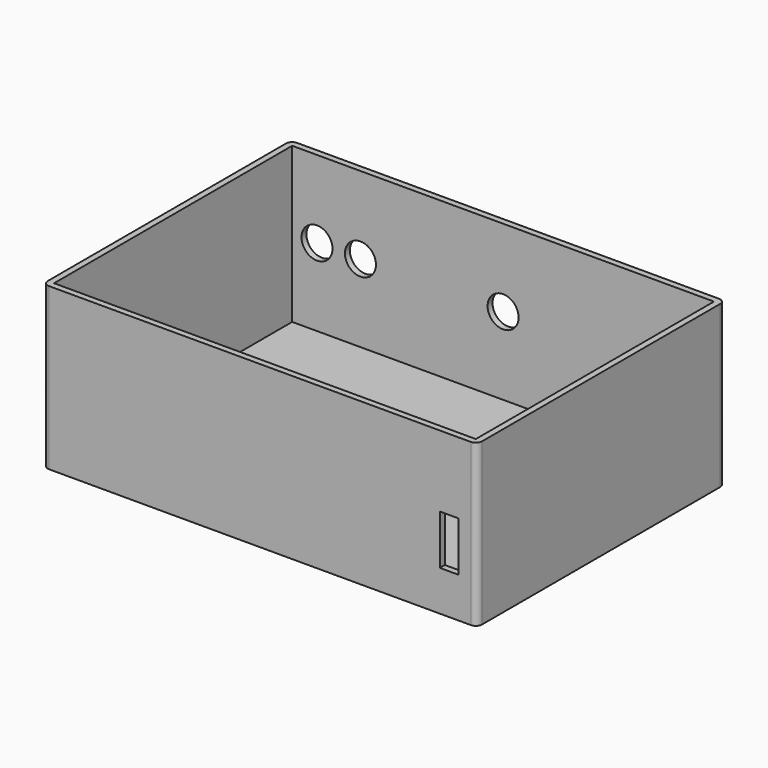
from build123d import *

# Parameters (mm, degrees)
F0_W          = 70
F0_H          = 50
F1_DEPTH      = 1
F2_W          = 70
F2_H          = 50
F2_W_2        = 68
F2_H_2        = 48
F3_DEPTH      = 25
F4_R          = 1
F5_W          = 3
F5_H          = 8
F6_DEPTH      = 25
F7_W          = 5
F7_H          = 10
F8_DEPTH      = 25
F9_R          = 2.5
F10_DEPTH     = 25
F11_R         = 2.5
F12_DEPTH     = 25
F13_R         = 2.5
F14_DEPTH     = 25
F15_TEXT_SIZE = 6.9444444444
F16_DEPTH     = 0.5


# Not quite as in the source:
# - Text() gives the source's letters only with a copy of the font that has no kerning and outlines rounded to 1/6400 em; it was checked with that copy


with BuildPart() as f1:
    # F0 (on Top) → F1 (new body)
    with BuildSketch(Plane.XY):
        with Locations((0, -0.7945728756)):
            Rectangle(F0_W, F0_H)
    extrude(amount=F1_DEPTH)

    # F2 (on face) → F3 (join)
    with BuildSketch(Plane.XY.offset(1)):
        with Locations((0, -0.7945728756)):
            Rectangle(F2_W, F2_H)
        with Locations((0, -0.7945728756)):
            Rectangle(F2_W_2, F2_H_2, mode=Mode.SUBTRACT)
    extrude(amount=F3_DEPTH)

    # F4
    f4_edges = [f1.edges().sort_by_distance(p)[0] for p in [
        (-35, 24.205427, 13),
        (-35, -25.794573, 13),
        (35, 24.205427, 13),
        (35, -25.794573, 13),
    ]]
    fillet(f4_edges, radius=F4_R)

    # F5 (on face) → F6 (cut)
    with BuildSketch(Plane(origin=(0, -24.7945728756, 0), x_dir=(-1, 0, 0), z_dir=(0, 1, 0))):
        with Locations((-30.5, 10.5)):
            Rectangle(F5_W, F5_H)
    extrude(amount=-F6_DEPTH, mode=Mode.SUBTRACT)

    # F7 (on face) → F8 (cut)
    with BuildSketch(Plane.XY.offset(1)):
        with Locations((30.5, 17.2054271244)):
            Rectangle(F7_W, F7_H)
    extrude(amount=-F8_DEPTH, mode=Mode.SUBTRACT)

    # F9 (on face) → F10 (cut)
    with BuildSketch(Plane.XZ.offset(-23.2054271244)):
        with Locations((-30, 13.5)):
            Circle(F9_R)
        with Locations((-23, 13.5)):
            Circle(F9_R)
    extrude(amount=-F10_DEPTH, mode=Mode.SUBTRACT)

    # F11 (on face) → F12 (cut)
    with BuildSketch(Plane.XZ.offset(-23.2054271244)):
        with Locations((27, 13.5)):
            Circle(F11_R)
    extrude(amount=-F12_DEPTH, mode=Mode.SUBTRACT)

    # F13 (on face) → F14 (cut)
    with BuildSketch(Plane.XZ.offset(-23.2054271244)):
        with Locations((0, 13.5)):
            Circle(F13_R)
    extrude(amount=-F14_DEPTH, mode=Mode.SUBTRACT)

    # F15 (on face) → F16 (cut)
    with BuildSketch(Plane(origin=(0, 24.2054271244, 0), x_dir=(-1, 0, 0), z_dir=(0, 1, 0))):
        with Locations((-31.1475824888, 19.4587637458)):
            Text('ON', F15_TEXT_SIZE, font='Open Sans', text_align=(TextAlign.LEFT, TextAlign.BOTTOM))
    extrude(amount=-F16_DEPTH, mode=Mode.SUBTRACT)


solid = f1.part
